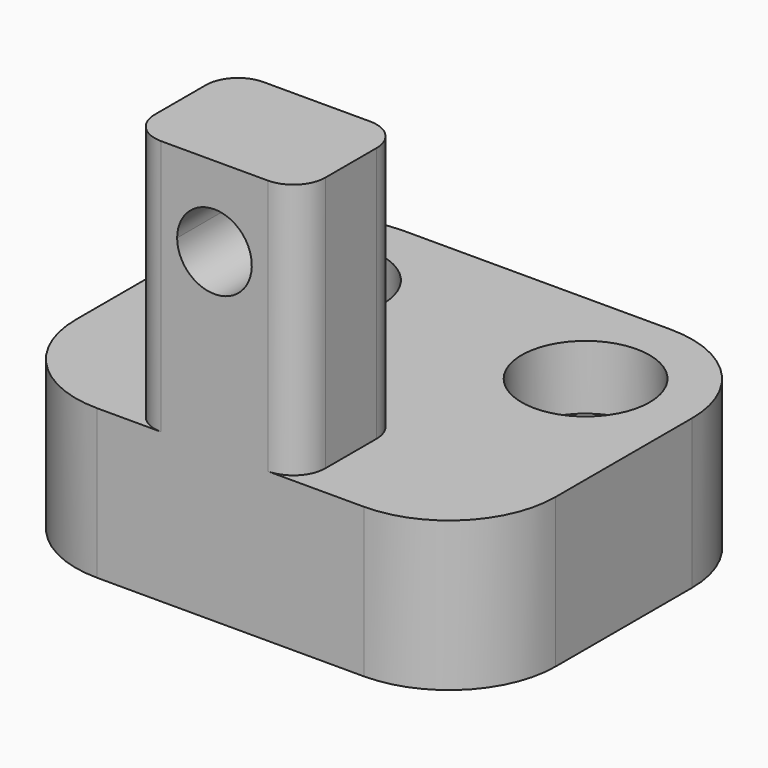
from build123d import *

# Parameters (mm, degrees)
F0_R      = 3
F0_R_2    = 1.75
F1_DEPTH  = 7
F3_DEPTH  = 5
F4_W      = 8
F4_H      = 6
F5_DEPTH  = 12
F6_R      = 1.5
F2_R      = 3
F2_R_2    = 1.75
F7_DEPTH  = 3
F8_R      = 5
F10_DEPTH = 25


# Not quite as in the source:
# - a feature names something its author has since deleted; it is built from what else it names


with BuildPart() as f1:
    # F0 (on Top) → F1 (new body)
    with BuildSketch(Plane.XY):
        with BuildLine():
            ThreePointArc((-51.1365796847, 36.9232990628), (-48.9174910641, 36.1016771789), (-47.9842549264, 33.9271686971))
            ThreePointArc((-47.9842549264, 33.9271686971), (-50.9842549264, 30.9271686971), (-53.9842549264, 33.9271686971))
            Line((-53.9842549264, 33.9271686971), (-55.9842549264, 33.9271686971))
            Line((-55.9842549264, 33.9271686971), (-55.9842549264, 28.9271686971))
            Line((-55.9842549264, 28.9271686971), (-35.9842549264, 28.9271686971))
            Line((-35.9842549264, 28.9271686971), (-35.9842549264, 25.9271686971))
            Line((-35.9842549264, 25.9271686971), (-33.4842549264, 25.9271686971))
            Line((-33.4842549264, 25.9271686971), (-33.4842549264, 33.9271686971))
            Line((-33.4842549264, 33.9271686971), (-33.4842549264, 38.9232990628))
            Line((-33.4842549264, 38.9232990628), (-35.9842549264, 38.9232990628))
            Line((-35.9842549264, 38.9232990628), (-51.1365796847, 38.9232990628))
            Line((-51.1365796847, 38.9232990628), (-51.1365796847, 36.9232990628))
        make_face()
        with Locations((-38.4842549264, 33.9271686971)):
            Circle(F0_R, mode=Mode.SUBTRACT)
        with BuildLine():
            ThreePointArc((-53.9842549264, 33.9271686971), (-53.1587634082, 35.9939325595), (-51.1365796847, 36.9232990628))
            Line((-51.1365796847, 36.9232990628), (-51.1365796847, 38.9232990628))
            Line((-51.1365796847, 38.9232990628), (-55.9842549264, 38.9232990628))
            Line((-55.9842549264, 38.9232990628), (-55.9842549264, 33.9271686971))
            Line((-55.9842549264, 33.9271686971), (-53.9842549264, 33.9271686971))
        make_face()
        Polygon((-35.9842549264, 28.9271686971), (-55.9842549264, 28.9271686971), (-55.9842549264, 25.9271686971), (-53.9842549264, 25.9271686971), (-43.9842549264, 25.9271686971), (-35.9842549264, 25.9271686971), align=None)
        with BuildLine():
            ThreePointArc((-53.9842549264, 33.9271686971), (-50.9842549264, 30.9271686971), (-47.9842549264, 33.9271686971))
            ThreePointArc((-47.9842549264, 33.9271686971), (-48.9174910641, 36.1016771789), (-51.1365796847, 36.9232990628))
            ThreePointArc((-51.1365796847, 36.9232990628), (-53.1587634082, 35.9939325595), (-53.9842549264, 33.9271686971))
        make_face()
        with Locations((-50.9842549264, 33.9271686971)):
            Circle(F0_R_2, mode=Mode.SUBTRACT)
        with Locations((-38.4842549264, 33.9271686971)):
            Circle(F0_R)
        with Locations((-38.4842549264, 33.9271686971)):
            Circle(F0_R_2, mode=Mode.SUBTRACT)
    extrude(amount=F1_DEPTH)

    # F3 (add): a face of the model
    f3_faces = [f1.faces().sort_by_distance(p)[0] for p in [
        (-44.7342549264, 25.9271686971, 3.5),
    ]]
    extrude(f3_faces, amount=F3_DEPTH)

    # F4 (on face) → F5 (join)
    with BuildSketch(Plane.XY.offset(7)):
        with Locations((-45.4842549264, 23.9271686971)):
            Rectangle(F4_W, F4_H)
    extrude(amount=F5_DEPTH)

    # F6
    f6_edges = [f1.edges().sort_by_distance(p)[0] for p in [
        (-49.484255, 20.927169, 13),
        (-41.484255, 20.927169, 13),
        (-49.484255, 26.927169, 13),
        (-41.484255, 26.927169, 13),
    ]]
    fillet(f6_edges, radius=F6_R)

    # F2 (on face) → F7 (cut)
    with BuildSketch(Plane.XY.offset(7)):
        with Locations((-50.9842549264, 33.9271686971)):
            Circle(F2_R)
        with Locations((-50.9842549264, 33.9271686971)):
            Circle(F2_R_2, mode=Mode.SUBTRACT)
        with Locations((-38.4842549264, 33.9271686971)):
            Circle(F2_R)
        with Locations((-38.4842549264, 33.9271686971)):
            Circle(F2_R_2, mode=Mode.SUBTRACT)
    extrude(amount=-F7_DEPTH, mode=Mode.SUBTRACT)

    # F8
    f8_edges = [f1.edges().sort_by_distance(p)[0] for p in [
        (-55.984255, 20.927169, 3.5),
        (-55.984255, 38.923299, 3.5),
        (-33.484255, 38.923299, 3.5),
        (-33.484255, 20.927169, 3.5),
    ]]
    fillet(f8_edges, radius=F8_R)

    # F9 (on face) → F10 (cut)
    with BuildSketch(Plane(origin=(0, 26.9271686971, 0), x_dir=(-1, 0, 0), z_dir=(0, 1, 0))):
        with BuildLine():
            ThreePointArc((45.4842549264, 17), (44.2468180594, 14.0125631329), (47.2342549264, 15.25))
            ThreePointArc((47.2342549264, 15.25), (46.7216917935, 16.4874368671), (45.4842549264, 17))
        make_face()
    extrude(amount=-F10_DEPTH, mode=Mode.SUBTRACT)


solid = f1.part
